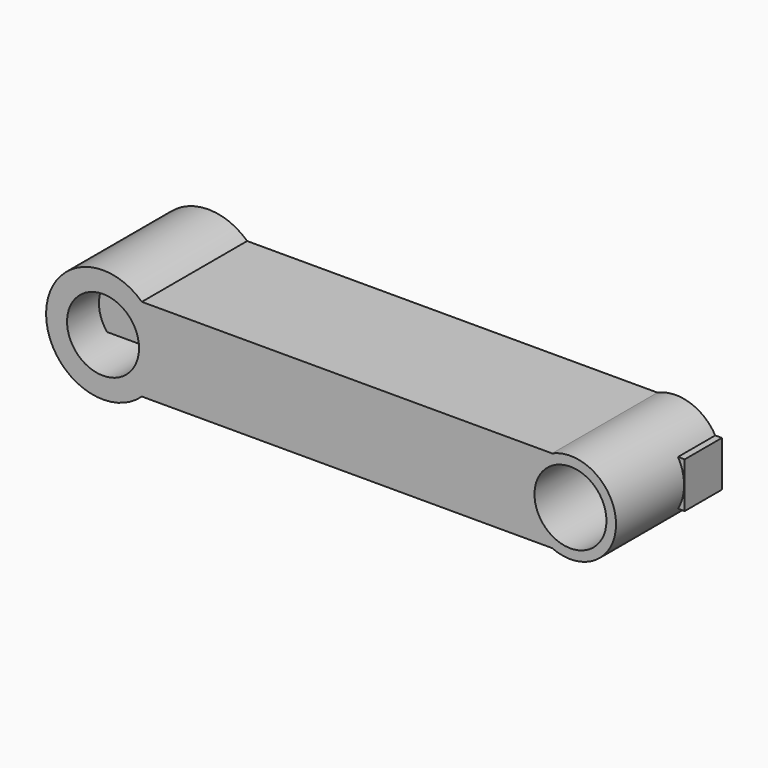
from build123d import *

# Parameters (mm, degrees)
F0_R     = 20.066
F1_DEPTH = 25.4
F2_DEPTH = 48.006
F3_W     = 1.0977562389
F3_H     = 41.91
F4_DEPTH = 12.7


with BuildPart() as f1:
    # F0 (on Front) → F1 (new body)
    with BuildSketch(Plane.XZ):
        with BuildLine():
            ThreePointArc((-10.2477275042, -23.241), (-25.4, 0), (-10.2477275042, 23.241))
            Line((-10.2477275042, 23.241), (-238.9725779709, 23.241))
            ThreePointArc((-238.9725779709, 23.241), (-231.493347745, 12.674084791), (-228.854, 0))
            ThreePointArc((-228.854, 0), (-231.493347745, -12.674084791), (-238.9725779709, -23.241))
            Line((-238.9725779709, -23.241), (-10.2477275042, -23.241))
        make_face()
        with BuildLine():
            ThreePointArc((-228.854, 0), (-231.493347745, 12.674084791), (-238.9725779709, 23.241))
            ThreePointArc((-238.9725779709, 23.241), (-292.354, 0), (-238.9725779709, -23.241))
            ThreePointArc((-238.9725779709, -23.241), (-231.493347745, -12.674084791), (-228.854, 0))
        make_face()
        with Locations((-260.604, 0)):
            Circle(F0_R, mode=Mode.SUBTRACT)
        with BuildLine():
            ThreePointArc((-10.2477275042, -23.241), (13.8720532257, -21.2773621322), (25.4, 0))
            ThreePointArc((25.4, 0), (13.8720532257, 21.2773621322), (-10.2477275042, 23.241))
            ThreePointArc((-10.2477275042, 23.241), (-25.4, 0), (-10.2477275042, -23.241))
        make_face()
        Circle(F0_R, mode=Mode.SUBTRACT)
    extrude(amount=F1_DEPTH)

    # F2 (add): a face of the model
    f2_faces = [f1.faces().sort_by_distance(p)[0] for p in [
        (-139.2710743105, -25.4, 0),
    ]]
    extrude(f2_faces, amount=F2_DEPTH)

    # F3 (on Top) → F4 (join, symmetric)
    with BuildSketch(Plane.XY):
        Polygon((-10.2477275042, 0), (-163.8780487135, 0), (-188.47713992, -9.2518740857), (-292.354, -9.2518740857), (-292.354, -51.1618740857), (-180.8564199804, -51.1618740857), (-113.8137692817, -25.9467083128), (-10.2477275042, -25.9467083128), align=None)
        Polygon((25.4, 0), (-10.2477275042, 0), (-10.2477275042, -25.9467083128), (25.713481009, -25.9467083128), (25.713481009, 0), align=None)
        with Locations((-292.9028781195, -30.2068740857)):
            Rectangle(F3_W, F3_H)
    extrude(amount=F4_DEPTH, both=True)


solid = f1.part
